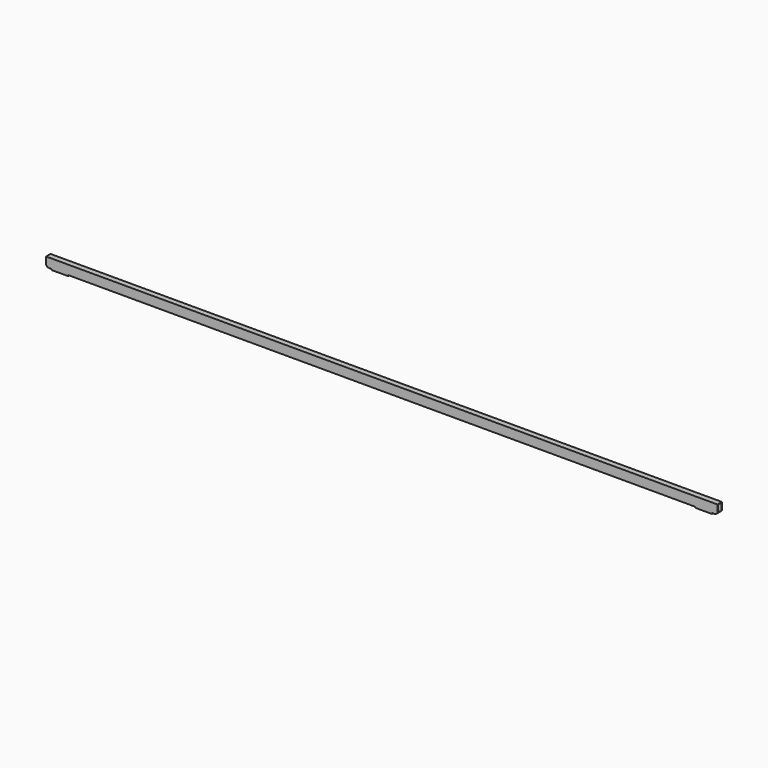
from build123d import *

# Parameters (mm, degrees)
F0_W          = 3575
F0_H          = 50
F1_DEPTH      = 15
F1_DEPTH_BACK = 15
F2_W          = 90
F2_H          = 30
F3_DEPTH      = 5
F4_W          = 90
F4_H          = 30
F5_DEPTH      = 5
F6_R          = 6
F7_DEPTH      = 25
F8_R          = 6
F9_DEPTH      = 5
F10_R         = 6
F11_DEPTH     = 5
F12_W         = 30
F12_H         = 50
F13_DEPTH     = 30
F14_R         = 15
F15_W         = 26
F15_H         = 13
F15_H_2       = 33
F16_DEPTH     = 100
F17_W         = 30
F17_H         = 50
F18_DEPTH     = 30
F19_W         = 26
F19_H         = 46
F20_DEPTH     = 100
F21_T1_DEPTH  = 105


# Not quite as in the source:
# - a fillet or chamfer that OpenCascade refuses, or shapes differently, is made with other operations: its cross-section is extruded or revolved along the edge and cut away or added


with BuildPart() as f1:
    # F0 (on Front) → F1 (new body, two sides)
    with BuildSketch(Plane.XZ) as f1_sk:
        Rectangle(F0_W, F0_H)
    extrude(amount=F1_DEPTH)
    extrude(f1_sk.sketch, amount=-F1_DEPTH_BACK)

    # F2 (on face) → F3 (join)
    with BuildSketch(Plane(origin=(0, 0, -25), x_dir=(1, 0, 0), z_dir=(0, 0, -1))):
        with Locations((-1742.5, -30)):
            Rectangle(F2_W, F2_H)
        Polygon((-1697.5, 15), (-1787.5, 15), (-1787.5, 0), (-1787.5, -15), (-1697.5, -15), align=None)
    extrude(amount=F3_DEPTH)

    # F4 (on face) → F5 (join)
    with BuildSketch(Plane(origin=(0, 0, -25), x_dir=(1, 0, 0), z_dir=(0, 0, -1))):
        with Locations((1742.5, -30)):
            Rectangle(F4_W, F4_H)
        Polygon((1787.5, 0), (1787.5, 15), (1697.5, 15), (1697.5, -15), (1787.5, -15), align=None)
    extrude(amount=F5_DEPTH)

    # F6 (on face) → F7 (cut, through all)
    with BuildSketch(Plane.XY):
        with Locations((-935, 30)):
            Circle(F6_R)
        with Locations((-975, 30)):
            Circle(F6_R)
    extrude(amount=-F7_DEPTH, mode=Mode.SUBTRACT)

    # F8 (on face) → F9 (cut, through all)
    with BuildSketch(Plane(origin=(0, 0, -30), x_dir=(1, 0, 0), z_dir=(0, 0, -1))):
        with Locations((1762.5, -30)):
            Circle(F8_R)
        with Locations((1722.5, -30)):
            Circle(F8_R)
    extrude(amount=-F9_DEPTH, mode=Mode.SUBTRACT)

    # F10 (on face) → F11 (cut, through all)
    with BuildSketch(Plane(origin=(0, 0, -30), x_dir=(1, 0, 0), z_dir=(0, 0, -1))):
        with Locations((-1722.5, -30)):
            Circle(F10_R)
        with Locations((-1762.5, -30)):
            Circle(F10_R)
    extrude(amount=-F11_DEPTH, mode=Mode.SUBTRACT)

    # F12 (on face) → F13 (join)
    with BuildSketch(Plane.YZ.offset(1787.5)):
        Rectangle(F12_W, F12_H)
    extrude(amount=F13_DEPTH)

    # F14
    f14_edges = [f1.edges().sort_by_distance(p)[0] for p in [
        (1817.5, 0, -25),
    ]]
    fillet(f14_edges, radius=F14_R)

    # F15 (on face) → F16 (cut)
    with BuildSketch(Plane.YZ.offset(1817.5)):
        with Locations((0, -16.5)):
            Rectangle(F15_W, F15_H)
        with Locations((0, 6.5)):
            Rectangle(F15_W, F15_H_2)
    extrude(amount=-F16_DEPTH, mode=Mode.SUBTRACT)

    # F17 (on face) → F18 (join)
    with BuildSketch(Plane(origin=(-1787.5, 0, 0), x_dir=(0, -1, 0), z_dir=(-1, 0, 0))):
        Rectangle(F17_W, F17_H)
    extrude(amount=F18_DEPTH)

    # F19 (on face) → F20 (cut)
    with BuildSketch(Plane(origin=(-1817.5, 0, 0), x_dir=(0, -1, 0), z_dir=(-1, 0, 0))):
        Rectangle(F19_W, F19_H)
    extrude(amount=-F20_DEPTH, mode=Mode.SUBTRACT)

    # F21: fillet of radius 15 on 1 edges, made by hand

    # F21_s2 → F21_t1 (cut)
    with BuildSketch(Plane.XZ.offset(-52.5)):
        with BuildLine():
            ThreePointArc((-1817.5, -10), (-1813.1066017178, -20.6066017178), (-1802.5, -25))
            Line((-1802.5, -25), (-1817.5, -25))
            Line((-1817.5, -25), (-1817.5, -10))
        make_face()
    extrude(amount=F21_T1_DEPTH, mode=Mode.SUBTRACT)


solid = f1.part
